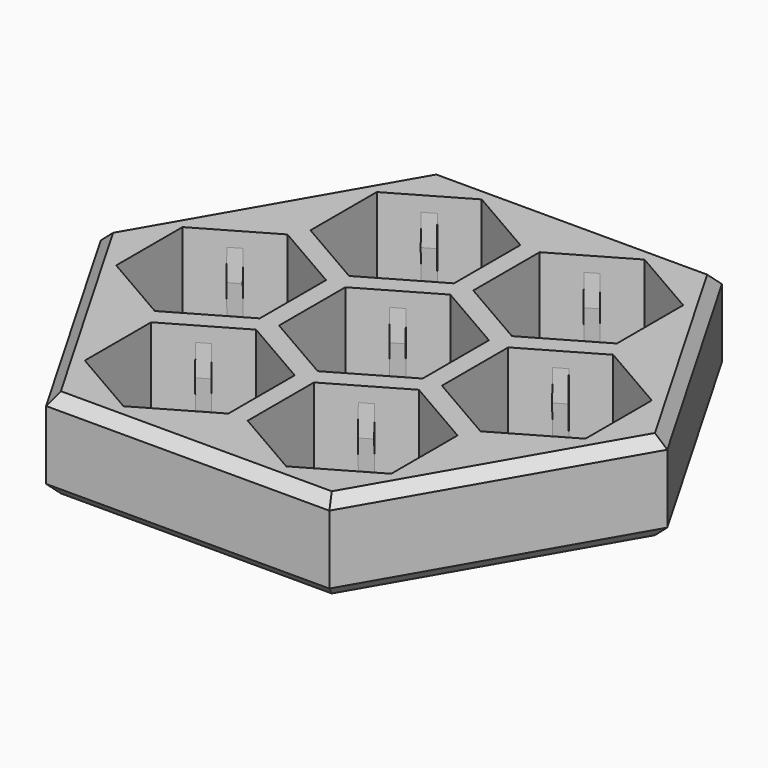
from build123d import *

# Parameters (mm, degrees)
F1_DEPTH    = 21
F2_SIZE     = 2.5
F3_W        = 3
F3_H        = 14
F4_DEPTH    = 0.5
F5_SIZE2    = 0.49999
F5_SIZE     = 6.99999
F6_W        = 3
F6_H        = 14
F7_DEPTH    = 0.5
F8_SIZE2    = 0.49999
F8_SIZE     = 6.99999
F8_2_SIZE2  = 0.49999
F8_2_SIZE   = 6.99999
F9_SIZE2    = 0.49999
F9_SIZE     = 6.99999
F10_W       = 3
F10_H       = 14
F11_DEPTH   = 0.5
F12_SIZE2   = 0.49999
F12_SIZE    = 6.99999
F13_W       = 3
F13_H       = 14
F14_DEPTH   = 0.5
F15_SIZE2   = 0.49999
F15_SIZE    = 6.99999
F15_2_SIZE2 = 0.49999
F15_2_SIZE  = 6.99999
F16_SIZE2   = 0.49999
F16_SIZE    = 6.99999
F17_W       = 3
F17_H       = 14
F18_DEPTH   = 0.5
F19_SIZE2   = 0.49999
F19_SIZE    = 6.99999
F20_W       = 3
F20_H       = 14
F21_DEPTH   = 0.5
F22_SIZE2   = 0.49999
F22_SIZE    = 6.99999
F23_W       = 3
F23_H       = 14
F24_DEPTH   = 0.5
F25_SIZE2   = 0.49999
F25_SIZE    = 6.99999
F25_2_SIZE2 = 0.49999
F25_2_SIZE  = 6.99999
F26_SIZE2   = 0.49999
F26_SIZE    = 6.99999
F27_W       = 3
F27_H       = 14
F28_DEPTH   = 0.5
F29_SIZE2   = 0.49999
F29_SIZE    = 6.99999
F30_W       = 3
F30_H       = 14
F31_DEPTH   = 0.5
F32_SIZE2   = 0.49999
F32_SIZE    = 6.99999
F32_2_SIZE2 = 0.49999
F32_2_SIZE  = 6.99999
F33_SIZE2   = 0.49999
F33_SIZE    = 6.99999
F34_W       = 3
F34_H       = 14
F35_DEPTH   = 0.5
F36_SIZE2   = 0.49999
F36_SIZE    = 6.99999
F37_W       = 3
F37_H       = 14
F38_DEPTH   = 0.5
F39_SIZE2   = 0.49999
F39_SIZE    = 6.99999
F40_W       = 3
F40_H       = 14
F41_DEPTH   = 0.5
F42_SIZE2   = 0.49999
F42_SIZE    = 6.99999
F42_2_SIZE2 = 0.49999
F42_2_SIZE  = 6.99999
F43_SIZE2   = 0.49999
F43_SIZE    = 6.99999
F44_W       = 3
F44_H       = 14
F45_DEPTH   = 0.5
F46_SIZE2   = 0.49999
F46_SIZE    = 6.99999
F47_W       = 3
F47_H       = 14
F48_DEPTH   = 0.5
F49_SIZE2   = 0.49999
F49_SIZE    = 6.99999
F49_2_SIZE2 = 0.49999
F49_2_SIZE  = 6.99999
F50_SIZE2   = 0.49999
F50_SIZE    = 6.99999
F51_W       = 3
F51_H       = 14
F52_DEPTH   = 0.5
F53_SIZE2   = 0.49999
F53_SIZE    = 6.99999


# Not quite as in the source:
# - a fillet or chamfer is up to 0.001 mm smaller than in the source, because OpenCascade refuses the exact size


with BuildPart() as f1:
    # F0 (on Top) → F1 (new body)
    with BuildSketch(Plane.XY):
        Polygon((66.1066058222, 0), (33.0533029111, 57.25), (-33.0533029111, 57.25), (-66.1066058222, 0), (-33.0533029111, -57.25), (33.0533029111, -57.25), align=None)
        Polygon((-19, -13.567731326), (-2.25, -23.2383483349), (-2.25, -42.5795823527), (-19, -52.2501993617), (-35.75, -42.5795823527), (-35.75, -23.2383483349), align=None, mode=Mode.SUBTRACT)
        Polygon((19, -13.567731326), (35.75, -23.2383483349), (35.75, -42.5795823527), (19, -52.2501993617), (2.25, -42.5795823527), (2.25, -23.2383483349), align=None, mode=Mode.SUBTRACT)
        Polygon((38, 19.3412340179), (54.75, 9.6706170089), (54.75, -9.6706170089), (38, -19.3412340179), (21.25, -9.6706170089), (21.25, 9.6706170089), align=None, mode=Mode.SUBTRACT)
        Polygon((-38, 19.3412340179), (-21.25, 9.6706170089), (-21.25, -9.6706170089), (-38, -19.3412340179), (-54.75, -9.6706170089), (-54.75, 9.6706170089), align=None, mode=Mode.SUBTRACT)
        Polygon((-19, 52.2501993617), (-2.25, 42.5795823527), (-2.25, 23.2383483349), (-19, 13.567731326), (-35.75, 23.2383483349), (-35.75, 42.5795823527), align=None, mode=Mode.SUBTRACT)
        Polygon((0, 19.3412340179), (16.75, 9.6706170089), (16.75, -9.6706170089), (0, -19.3412340179), (-16.75, -9.6706170089), (-16.75, 9.6706170089), align=None, mode=Mode.SUBTRACT)
        Polygon((19, 52.2501993617), (35.75, 42.5795823527), (35.75, 23.2383483349), (19, 13.567731326), (2.25, 23.2383483349), (2.25, 42.5795823527), align=None, mode=Mode.SUBTRACT)
    extrude(amount=F1_DEPTH)

    # F2
    f2_edges = [f1.edges().sort_by_distance(p)[0] for p in [
        (0, 57.25, 21),
        (-49.579954, 28.625, 21),
        (-49.579954, -28.625, 21),
        (0, -57.25, 21),
        (49.579954, -28.625, 21),
        (49.579954, 28.625, 21),
        (49.579954, -28.625, 0),
        (0, -57.25, 0),
        (49.579954, 28.625, 0),
        (0, 57.25, 0),
        (-49.579954, 28.625, 0),
        (-49.579954, -28.625, 0),
    ]]
    chamfer(f2_edges, length=F2_SIZE)

    # F3 (on face) → F4 (join)
    with BuildSketch(Plane(origin=(-27.375, 47.4148908572, 0), x_dir=(0.8660254038, 0.5, 0), z_dir=(0.5, -0.8660254038, 0))):
        with Locations((0, 10.5)):
            Rectangle(F3_W, F3_H)
    extrude(amount=F4_DEPTH)

    # F5 (size 7 and 0.5 in the source; OpenCascade refuses exactly that, so slightly less here)
    f5_edges = [f1.edges().sort_by_distance(p)[0] for p in [
        (-27.125, 46.981878, 17.5),
        (-27.125, 46.981878, 3.5),
    ]]
    f5_side = f1.faces().sort_by_distance((-27.125, 46.981878, 10.5))[0]
    chamfer(f5_edges, length=F5_SIZE, length2=F5_SIZE2, reference=f5_side)

    # F6 (on face) → F7 (join)
    with BuildSketch(Plane(origin=(-17.875, 30.9604081853, 0), x_dir=(0.8660254038, 0.5, 0), z_dir=(0.5, -0.8660254038, 0))):
        with Locations((32.9088483349, 10.5)):
            Rectangle(F6_W, F6_H)
        with Locations((-32.9090823527, 10.5)):
            Rectangle(F6_W, F6_H)
    extrude(amount=F7_DEPTH)

    # F8 (size 7 and 0.5 in the source; OpenCascade refuses exactly that, so slightly less here)
    f8_edges = [f1.edges().sort_by_distance(p)[0] for p in [
        (-46.125101, 14.072854, 17.5),
        (-46.125101, 14.072854, 3.5),
    ]]
    f8_side = f1.faces().sort_by_distance((-46.125101, 14.072854, 10.5))[0]
    chamfer(f8_edges, length=F8_SIZE, length2=F8_SIZE2, reference=f8_side)

    # F8#2 (size 7 and 0.5 in the source; OpenCascade refuses exactly that, so slightly less here)
    f8_2_edges = [f1.edges().sort_by_distance(p)[0] for p in [
        (10.874899, 46.98182, 17.5),
    ]]
    f8_2_side = f1.faces().sort_by_distance((10.874899, 46.98182, 10.5))[0]
    chamfer(f8_2_edges, length=F8_2_SIZE, length2=F8_2_SIZE2, reference=f8_2_side)

    # F9 (size 7 and 0.5 in the source; OpenCascade refuses exactly that, so slightly less here)
    f9_edges = [f1.edges().sort_by_distance(p)[0] for p in [
        (10.874899, 46.98182, 3.5),
    ]]
    f9_side = f1.faces().sort_by_distance((10.874899, 46.98182, 7.000005))[0]
    chamfer(f9_edges, length=F9_SIZE, length2=F9_SIZE2, reference=f9_side)

    # F10 (on face) → F11 (join)
    with BuildSketch(Plane(origin=(-8.375, 14.5059255134, 0), x_dir=(0.8660254038, 0.5, 0), z_dir=(0.5, -0.8660254038, 0))):
        with Locations((0, 10.5)):
            Rectangle(F10_W, F10_H)
    extrude(amount=F11_DEPTH)

    # F12 (size 7 and 0.5 in the source; OpenCascade refuses exactly that, so slightly less here)
    f12_edges = [f1.edges().sort_by_distance(p)[0] for p in [
        (-8.125, 14.072913, 17.5),
        (-8.125, 14.072913, 3.5),
    ]]
    f12_side = f1.faces().sort_by_distance((-8.125, 14.072913, 10.5))[0]
    chamfer(f12_edges, length=F12_SIZE, length2=F12_SIZE2, reference=f12_side)

    # F13 (on face) → F14 (join)
    with BuildSketch(Plane(origin=(1.125, -1.9485571585, 0), x_dir=(0.8660254038, 0.5, 0), z_dir=(0.5, -0.8660254038, 0))):
        with Locations((-32.9090823527, 10.5)):
            Rectangle(F13_W, F13_H)
        with Locations((32.9088483349, 10.5)):
            Rectangle(F13_W, F13_H)
    extrude(amount=F14_DEPTH)

    # F15 (size 7 and 0.5 in the source; OpenCascade refuses exactly that, so slightly less here)
    f15_edges = [f1.edges().sort_by_distance(p)[0] for p in [
        (-27.125101, -18.836111, 17.5),
        (-27.125101, -18.836111, 3.5),
    ]]
    f15_side = f1.faces().sort_by_distance((-27.125101, -18.836111, 10.5))[0]
    chamfer(f15_edges, length=F15_SIZE, length2=F15_SIZE2, reference=f15_side)

    # F15#2 (size 7 and 0.5 in the source; OpenCascade refuses exactly that, so slightly less here)
    f15_2_edges = [f1.edges().sort_by_distance(p)[0] for p in [
        (29.874899, 14.072854, 17.5),
    ]]
    f15_2_side = f1.faces().sort_by_distance((29.874899, 14.072854, 10.5))[0]
    chamfer(f15_2_edges, length=F15_2_SIZE, length2=F15_2_SIZE2, reference=f15_2_side)

    # F16 (size 7 and 0.5 in the source; OpenCascade refuses exactly that, so slightly less here)
    f16_edges = [f1.edges().sort_by_distance(p)[0] for p in [
        (29.874899, 14.072854, 3.5),
    ]]
    f16_side = f1.faces().sort_by_distance((29.874899, 14.072854, 7.000005))[0]
    chamfer(f16_edges, length=F16_SIZE, length2=F16_SIZE2, reference=f16_side)

    # F17 (on face) → F18 (join)
    with BuildSketch(Plane(origin=(10.625, -18.4030398304, 0), x_dir=(0.8660254038, 0.5, 0), z_dir=(0.5, -0.8660254038, 0))):
        with Locations((0, 10.5)):
            Rectangle(F17_W, F17_H)
    extrude(amount=F18_DEPTH)

    # F19 (size 7 and 0.5 in the source; OpenCascade refuses exactly that, so slightly less here)
    f19_edges = [f1.edges().sort_by_distance(p)[0] for p in [
        (10.875, -18.836053, 17.5),
        (10.875, -18.836053, 3.5),
    ]]
    f19_side = f1.faces().sort_by_distance((10.875, -18.836053, 10.5))[0]
    chamfer(f19_edges, length=F19_SIZE, length2=F19_SIZE2, reference=f19_side)

    # F20 (on face) → F21 (join)
    with BuildSketch(Plane(origin=(54.75, 0, 0), x_dir=(0, -1, 0), z_dir=(-1, 0, 0))):
        with Locations((0, 10.5)):
            Rectangle(F20_W, F20_H)
    extrude(amount=F21_DEPTH)

    # F22 (size 7 and 0.5 in the source; OpenCascade refuses exactly that, so slightly less here)
    f22_edges = [f1.edges().sort_by_distance(p)[0] for p in [
        (54.25, 0, 17.5),
        (54.25, 0, 3.5),
    ]]
    f22_side = f1.faces().sort_by_distance((54.25, 0, 10.5))[0]
    chamfer(f22_edges, length=F22_SIZE, length2=F22_SIZE2, reference=f22_side)

    # F23 (on face) → F24 (join)
    with BuildSketch(Plane(origin=(35.75, 0, 0), x_dir=(0, -1, 0), z_dir=(-1, 0, 0))):
        with Locations((-32.9090823527, 10.5)):
            Rectangle(F23_W, F23_H)
        with Locations((32.9088483349, 10.5)):
            Rectangle(F23_W, F23_H)
    extrude(amount=F24_DEPTH)

    # F25 (size 7 and 0.5 in the source; OpenCascade refuses exactly that, so slightly less here)
    f25_edges = [f1.edges().sort_by_distance(p)[0] for p in [
        (35.25, -32.908848, 17.5),
        (35.25, -32.908848, 3.5),
    ]]
    f25_side = f1.faces().sort_by_distance((35.25, -32.908848, 10.5))[0]
    chamfer(f25_edges, length=F25_SIZE, length2=F25_SIZE2, reference=f25_side)

    # F25#2 (size 7 and 0.5 in the source; OpenCascade refuses exactly that, so slightly less here)
    f25_2_edges = [f1.edges().sort_by_distance(p)[0] for p in [
        (35.25, 32.909082, 17.5),
    ]]
    f25_2_side = f1.faces().sort_by_distance((35.25, 32.909082, 10.5))[0]
    chamfer(f25_2_edges, length=F25_2_SIZE, length2=F25_2_SIZE2, reference=f25_2_side)

    # F26 (size 7 and 0.5 in the source; OpenCascade refuses exactly that, so slightly less here)
    f26_edges = [f1.edges().sort_by_distance(p)[0] for p in [
        (35.25, 32.909082, 3.5),
    ]]
    f26_side = f1.faces().sort_by_distance((35.25, 32.909082, 7.000005))[0]
    chamfer(f26_edges, length=F26_SIZE, length2=F26_SIZE2, reference=f26_side)

    # F27 (on face) → F28 (join)
    with BuildSketch(Plane(origin=(16.75, 0, 0), x_dir=(0, -1, 0), z_dir=(-1, 0, 0))):
        with Locations((0, 10.5)):
            Rectangle(F27_W, F27_H)
    extrude(amount=F28_DEPTH)

    # F29 (size 7 and 0.5 in the source; OpenCascade refuses exactly that, so slightly less here)
    f29_edges = [f1.edges().sort_by_distance(p)[0] for p in [
        (16.25, 0, 17.5),
        (16.25, 0, 3.5),
    ]]
    f29_side = f1.faces().sort_by_distance((16.25, 0, 10.5))[0]
    chamfer(f29_edges, length=F29_SIZE, length2=F29_SIZE2, reference=f29_side)

    # F30 (on face) → F31 (join)
    with BuildSketch(Plane(origin=(-2.25, 0, 0), x_dir=(0, -1, 0), z_dir=(-1, 0, 0))):
        with Locations((-32.9090823527, 10.5)):
            Rectangle(F30_W, F30_H)
        with Locations((32.9088483349, 10.5)):
            Rectangle(F30_W, F30_H)
    extrude(amount=F31_DEPTH)

    # F32 (size 7 and 0.5 in the source; OpenCascade refuses exactly that, so slightly less here)
    f32_edges = [f1.edges().sort_by_distance(p)[0] for p in [
        (-2.75, 32.909082, 17.5),
        (-2.75, 32.909082, 3.5),
    ]]
    f32_side = f1.faces().sort_by_distance((-2.75, 32.909082, 10.5))[0]
    chamfer(f32_edges, length=F32_SIZE, length2=F32_SIZE2, reference=f32_side)

    # F32#2 (size 7 and 0.5 in the source; OpenCascade refuses exactly that, so slightly less here)
    f32_2_edges = [f1.edges().sort_by_distance(p)[0] for p in [
        (-2.75, -32.908848, 17.5),
    ]]
    f32_2_side = f1.faces().sort_by_distance((-2.75, -32.908848, 10.5))[0]
    chamfer(f32_2_edges, length=F32_2_SIZE, length2=F32_2_SIZE2, reference=f32_2_side)

    # F33 (size 7 and 0.5 in the source; OpenCascade refuses exactly that, so slightly less here)
    f33_edges = [f1.edges().sort_by_distance(p)[0] for p in [
        (-2.75, -32.908848, 3.5),
    ]]
    f33_side = f1.faces().sort_by_distance((-2.75, -32.908848, 7.000005))[0]
    chamfer(f33_edges, length=F33_SIZE, length2=F33_SIZE2, reference=f33_side)

    # F34 (on face) → F35 (join)
    with BuildSketch(Plane(origin=(-21.25, 0, 0), x_dir=(0, -1, 0), z_dir=(-1, 0, 0))):
        with Locations((0, 10.5)):
            Rectangle(F34_W, F34_H)
    extrude(amount=F35_DEPTH)

    # F36 (size 7 and 0.5 in the source; OpenCascade refuses exactly that, so slightly less here)
    f36_edges = [f1.edges().sort_by_distance(p)[0] for p in [
        (-21.75, 0, 17.5),
        (-21.75, 0, 3.5),
    ]]
    f36_side = f1.faces().sort_by_distance((-21.75, 0, 10.5))[0]
    chamfer(f36_edges, length=F36_SIZE, length2=F36_SIZE2, reference=f36_side)

    # F37 (on face) → F38 (join)
    with BuildSketch(Plane(origin=(-27.375, -47.4148908572, 0), x_dir=(-0.8660254038, 0.5, 0), z_dir=(0.5, 0.8660254038, 0))):
        with Locations((0, 10.5)):
            Rectangle(F37_W, F37_H)
    extrude(amount=F38_DEPTH)

    # F39 (size 7 and 0.5 in the source; OpenCascade refuses exactly that, so slightly less here)
    f39_edges = [f1.edges().sort_by_distance(p)[0] for p in [
        (-27.125, -46.981878, 17.5),
        (-27.125, -46.981878, 3.5),
    ]]
    f39_side = f1.faces().sort_by_distance((-27.125, -46.981878, 10.5))[0]
    chamfer(f39_edges, length=F39_SIZE, length2=F39_SIZE2, reference=f39_side)

    # F40 (on face) → F41 (join)
    with BuildSketch(Plane(origin=(-17.875, -30.9604081853, 0), x_dir=(-0.8660254038, 0.5, 0), z_dir=(0.5, 0.8660254038, 0))):
        with Locations((-32.9090823527, 10.5)):
            Rectangle(F40_W, F40_H)
        with Locations((32.9088483349, 10.5)):
            Rectangle(F40_W, F40_H)
    extrude(amount=F41_DEPTH)

    # F42 (size 7 and 0.5 in the source; OpenCascade refuses exactly that, so slightly less here)
    f42_edges = [f1.edges().sort_by_distance(p)[0] for p in [
        (10.875101, -46.981937, 17.5),
        (10.875101, -46.981937, 3.5),
    ]]
    f42_side = f1.faces().sort_by_distance((10.875101, -46.981937, 10.5))[0]
    chamfer(f42_edges, length=F42_SIZE, length2=F42_SIZE2, reference=f42_side)

    # F42#2 (size 7 and 0.5 in the source; OpenCascade refuses exactly that, so slightly less here)
    f42_2_edges = [f1.edges().sort_by_distance(p)[0] for p in [
        (-46.124899, -14.072971, 17.5),
    ]]
    f42_2_side = f1.faces().sort_by_distance((-46.124899, -14.072971, 10.5))[0]
    chamfer(f42_2_edges, length=F42_2_SIZE, length2=F42_2_SIZE2, reference=f42_2_side)

    # F43 (size 7 and 0.5 in the source; OpenCascade refuses exactly that, so slightly less here)
    f43_edges = [f1.edges().sort_by_distance(p)[0] for p in [
        (-46.124899, -14.072971, 3.5),
    ]]
    f43_side = f1.faces().sort_by_distance((-46.124899, -14.072971, 7.000005))[0]
    chamfer(f43_edges, length=F43_SIZE, length2=F43_SIZE2, reference=f43_side)

    # F44 (on face) → F45 (join)
    with BuildSketch(Plane(origin=(-8.375, -14.5059255134, 0), x_dir=(-0.8660254038, 0.5, 0), z_dir=(0.5, 0.8660254038, 0))):
        with Locations((0, 10.5)):
            Rectangle(F44_W, F44_H)
    extrude(amount=F45_DEPTH)

    # F46 (size 7 and 0.5 in the source; OpenCascade refuses exactly that, so slightly less here)
    f46_edges = [f1.edges().sort_by_distance(p)[0] for p in [
        (-8.125, -14.072913, 17.5),
        (-8.125, -14.072913, 3.5),
    ]]
    f46_side = f1.faces().sort_by_distance((-8.125, -14.072913, 10.5))[0]
    chamfer(f46_edges, length=F46_SIZE, length2=F46_SIZE2, reference=f46_side)

    # F47 (on face) → F48 (join)
    with BuildSketch(Plane(origin=(1.125, 1.9485571585, 0), x_dir=(-0.8660254038, 0.5, 0), z_dir=(0.5, 0.8660254038, 0))):
        with Locations((-32.9090823527, 10.5)):
            Rectangle(F47_W, F47_H)
        with Locations((32.9088483349, 10.5)):
            Rectangle(F47_W, F47_H)
    extrude(amount=F48_DEPTH)

    # F49 (size 7 and 0.5 in the source; OpenCascade refuses exactly that, so slightly less here)
    f49_edges = [f1.edges().sort_by_distance(p)[0] for p in [
        (-27.124899, 18.835994, 17.5),
        (-27.124899, 18.835994, 3.5),
    ]]
    f49_side = f1.faces().sort_by_distance((-27.124899, 18.835994, 10.5))[0]
    chamfer(f49_edges, length=F49_SIZE, length2=F49_SIZE2, reference=f49_side)

    # F49#2 (size 7 and 0.5 in the source; OpenCascade refuses exactly that, so slightly less here)
    f49_2_edges = [f1.edges().sort_by_distance(p)[0] for p in [
        (29.875101, -14.072971, 17.5),
    ]]
    f49_2_side = f1.faces().sort_by_distance((29.875101, -14.072971, 10.5))[0]
    chamfer(f49_2_edges, length=F49_2_SIZE, length2=F49_2_SIZE2, reference=f49_2_side)

    # F50 (size 7 and 0.5 in the source; OpenCascade refuses exactly that, so slightly less here)
    f50_edges = [f1.edges().sort_by_distance(p)[0] for p in [
        (29.875101, -14.072971, 3.5),
    ]]
    f50_side = f1.faces().sort_by_distance((29.875101, -14.072971, 7.000005))[0]
    chamfer(f50_edges, length=F50_SIZE, length2=F50_SIZE2, reference=f50_side)

    # F51 (on face) → F52 (join)
    with BuildSketch(Plane(origin=(10.625, 18.4030398304, 0), x_dir=(-0.8660254038, 0.5, 0), z_dir=(0.5, 0.8660254038, 0))):
        with Locations((0, 10.5)):
            Rectangle(F51_W, F51_H)
    extrude(amount=F52_DEPTH)

    # F53 (size 7 and 0.5 in the source; OpenCascade refuses exactly that, so slightly less here)
    f53_edges = [f1.edges().sort_by_distance(p)[0] for p in [
        (10.875, 18.836053, 17.5),
        (10.875, 18.836053, 3.5),
    ]]
    f53_side = f1.faces().sort_by_distance((10.875, 18.836053, 10.5))[0]
    chamfer(f53_edges, length=F53_SIZE, length2=F53_SIZE2, reference=f53_side)


solid = f1.part
